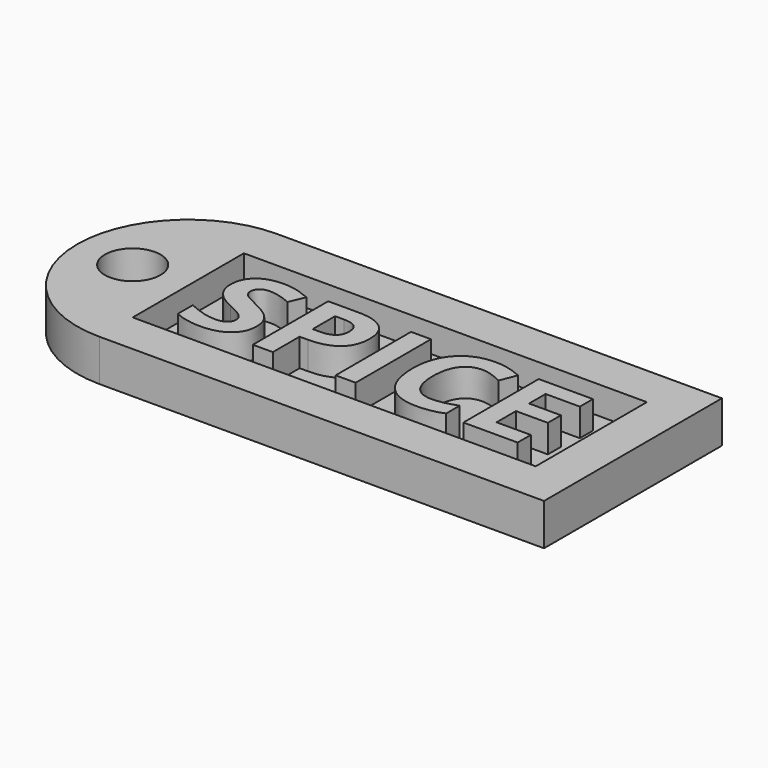
from build123d import *

# Parameters (mm, degrees)
F1_DEPTH     = 3.81
F2_W         = 36.83
F2_H         = 12.7
F3_DEPTH     = 2.54
F4_R         = 2.54
F5_DEPTH     = 25.4
F6_TEXT_SIZE = 12.0536411285
F7_DEPTH     = 2.54


# Not quite as in the source:
# - Text() gives the source's letters only with a copy of the font that has no kerning and outlines rounded to 1/6400 em; it was checked with that copy


with BuildPart() as f1:
    # F0 (on Top) → F1 (new body)
    with BuildSketch(Plane.XY):
        with BuildLine():
            Line((32.3745887542, 25.9258832581), (-8.2654112458, 25.9258832581))
            ThreePointArc((-8.2654112458, 25.9258832581), (-15.4496161427, 22.9500881549), (-18.4254112458, 15.7658832581))
            ThreePointArc((-18.4254112458, 15.7658832581), (-15.4496161427, 8.5816783612), (-8.2654112458, 5.6058832581))
            Line((-8.2654112458, 5.6058832581), (32.3745887542, 5.6058832581))
            Line((32.3745887542, 5.6058832581), (32.3745887542, 25.9258832581))
        make_face()
    extrude(amount=F1_DEPTH)

    # F2 (on face) → F3 (cut)
    with BuildSketch(Plane.XY.offset(3.81)):
        with Locations((10.1495887542, 15.7658832581)):
            Rectangle(F2_W, F2_H)
    extrude(amount=-F3_DEPTH, mode=Mode.SUBTRACT)

    # F4 (on face) → F5 (cut)
    with BuildSketch(Plane.XY.offset(3.81)):
        with Locations((-13.3454112458, 15.7658832581)):
            Circle(F4_R)
    extrude(amount=-F5_DEPTH, mode=Mode.SUBTRACT)

    # F6 (on face) → F7 (join)
    with BuildSketch(Plane.XY.offset(1.27)):
        with Locations((-6.6553880461, 11.4773483947)):
            Text('SPICE', F6_TEXT_SIZE, font='Open Sans', font_style=FontStyle.BOLD, text_align=(TextAlign.LEFT, TextAlign.BOTTOM))
    extrude(amount=F7_DEPTH)


solid = f1.part
